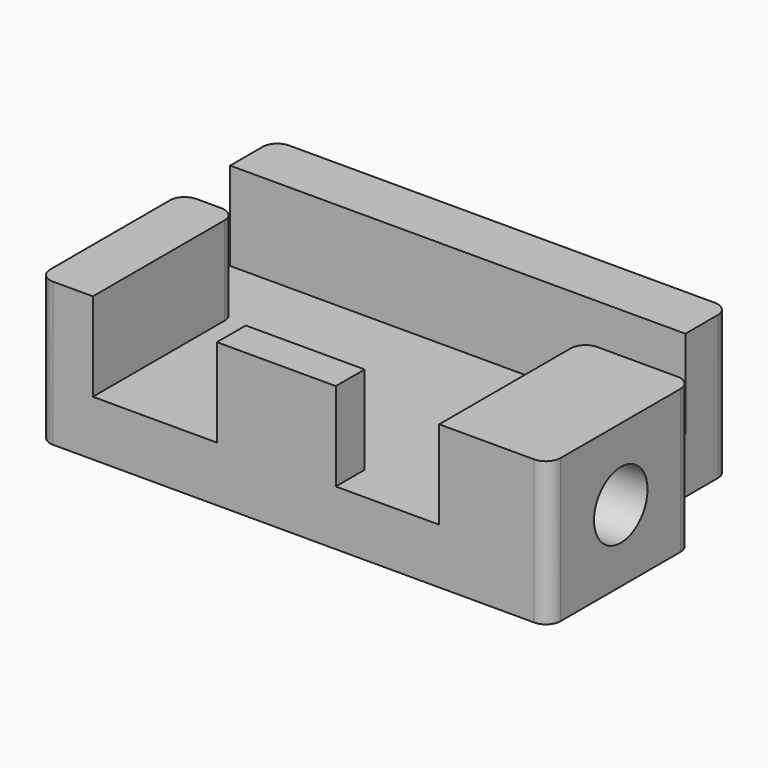
from build123d import *

# Parameters (mm, degrees)
F0_W     = 39.243
F0_H     = 25.4254
F1_DEPTH = 4.7625
F2_W     = 4.69392
F2_H     = 15.4432
F2_W_2   = 10.2489
F2_H_2   = 3.1115
F2_W_3   = 39.243
F2_H_3   = 4.7625
F3_DEPTH = 7.62
F5_DEPTH = 4.7625
F7_D     = 5.7658
F7_DEPTH = 4.7625
F7_TIP   = 1.7322210786
F8_R     = 1.27


# Not quite as in the source:
# - a length typed as a fraction of an inch, garbled in the dataset ("3 / 203.2 mm" for 3/8 in), is restored


with BuildPart() as f1:
    # F0 (on Top) → F1 (new body)
    with BuildSketch(Plane.XY):
        Rectangle(F0_W, F0_H)
    extrude(amount=F1_DEPTH)

    # F2 (on face) → F3 (join)
    with BuildSketch(Plane.XY.offset(4.7625)):
        with Locations((-17.27454, -4.9911)):
            Rectangle(F2_W, F2_H)
        with Locations((17.27454, -4.9911)):
            Rectangle(F2_W, F2_H)
        with Locations((0.89027, -11.15695)):
            Rectangle(F2_W_2, F2_H_2)
        with Locations((0, 10.33145)):
            Rectangle(F2_W_3, F2_H_3)
    extrude(amount=F3_DEPTH)

    # F4 (on face) → F5 (join)
    with BuildSketch(Plane.YZ.offset(19.6215)):
        Polygon((2.7305, 4.7625), (2.7305, 12.3825), (-12.7127, 12.3825), (-12.7127, 0), (2.7305, 0), align=None)
    extrude(amount=F5_DEPTH)

    # F7
    with Locations(Plane.YZ.offset(24.384)):
        with Locations((-4.9657, 6.19125)):
            Hole(F7_D / 2, depth=F7_DEPTH)
            with Locations((0, 0, -(F7_DEPTH + F7_TIP / 2))):  # 118° drill point
                Cone(0, F7_D / 2, F7_TIP, mode=Mode.SUBTRACT)

    # F8
    f8_edges = [f1.edges().sort_by_distance(p)[0] for p in [
        (-14.92758, 2.7305, 8.5725),
        (14.92758, 2.7305, 8.5725),
        (-19.6215, -12.7127, 6.19125),
        (24.384, -12.7127, 6.19125),
        (24.384, 2.7305, 6.19125),
        (19.6215, 12.7127, 6.19125),
        (-19.6215, 12.7127, 6.19125),
        (-19.6215, 2.7305, 8.5725),
    ]]
    fillet(f8_edges, radius=F8_R)


solid = f1.part
